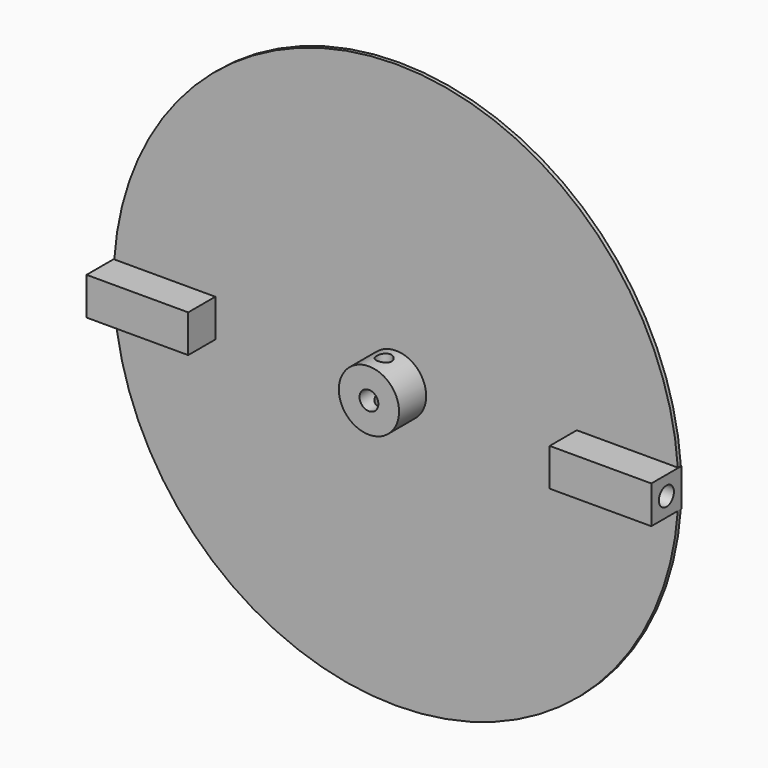
from build123d import *

# Parameters (mm, degrees)
F0_W          = 27
F0_H          = 10
F1_DEPTH      = 10
F0_R          = 2.5
F2_R          = 75
F2_R_2        = 2.5
F3_DEPTH      = 1
F4_R          = 2.5
F5_DEPTH      = 25
F6_R          = 2
F7_DEPTH      = 75.001
F7_DEPTH_BACK = 75.001


# Not quite as in the source:
# - a pattern or mirror of a feature is missing from the dataset's text; its kind, count and spacing are read off the source's solid


with BuildPart() as f1:
    # F0 (on Front) → F1 (new body)
    with BuildSketch(Plane.XZ):
        with Locations((61.5, 0)):
            Rectangle(F0_W, F0_H)
    extrude(amount=F1_DEPTH)



with BuildPart() as f1b:
    # F0 (on Front) → F1, piece 2 (new body)
    with BuildSketch(Plane.XZ):
        with Locations((-61.5, 0)):
            Rectangle(F0_W, F0_H)
    extrude(amount=F1_DEPTH)


with BuildPart() as f1c:
    # F0 (on Front) → F1, piece 3 (new body)
    with BuildSketch(Plane.XZ):
        with BuildLine():
            ThreePointArc((6.2449979984, 5), (0, 8), (-6.2449979984, 5))
            ThreePointArc((-6.2449979984, 5), (-8, 0), (-6.2449979984, -5))
            ThreePointArc((-6.2449979984, -5), (0, -8), (6.2449979984, -5))
            ThreePointArc((6.2449979984, -5), (8, 0), (6.2449979984, 5))
        make_face()
        Circle(F0_R, mode=Mode.SUBTRACT)
    extrude(amount=F1_DEPTH)


with BuildPart() as f1_1:
    add(f1.part)

    add(f1b.part)  # F3 merges F1b

    add(f1c.part)  # F3 merges F1c
    # F2 (on face) → F3 (join)
    with BuildSketch(Plane(origin=(0, 0, 0), x_dir=(-1, 0, 0), z_dir=(0, 1, 0))):
        Circle(F2_R)
        Circle(F2_R_2, mode=Mode.SUBTRACT)
    extrude(amount=-F3_DEPTH)

    # F4 (on face) → F5 (cut)
    with BuildSketch(Plane(origin=(-75, 0, 0), x_dir=(0, -1, 0), z_dir=(-1, 0, 0))):
        with Locations((5, 0)):
            Circle(F4_R)
    f5 = extrude(amount=-F5_DEPTH, mode=Mode.SUBTRACT)

    # F5_copies: F5 across plane
    add(f5.mirror(Plane(origin=(0, 0, 0), x_dir=(0, 0, 1), z_dir=(1, 0, 0))), mode=Mode.SUBTRACT)

    # F6 (on Top) → F7 (cut, two sides)
    with BuildSketch(Plane.XY) as f7_sk:
        with Locations((0, -5)):
            Circle(F6_R)
    extrude(amount=-F7_DEPTH, mode=Mode.SUBTRACT)
    extrude(f7_sk.sketch, amount=F7_DEPTH_BACK, mode=Mode.SUBTRACT)


solid = f1_1.part
